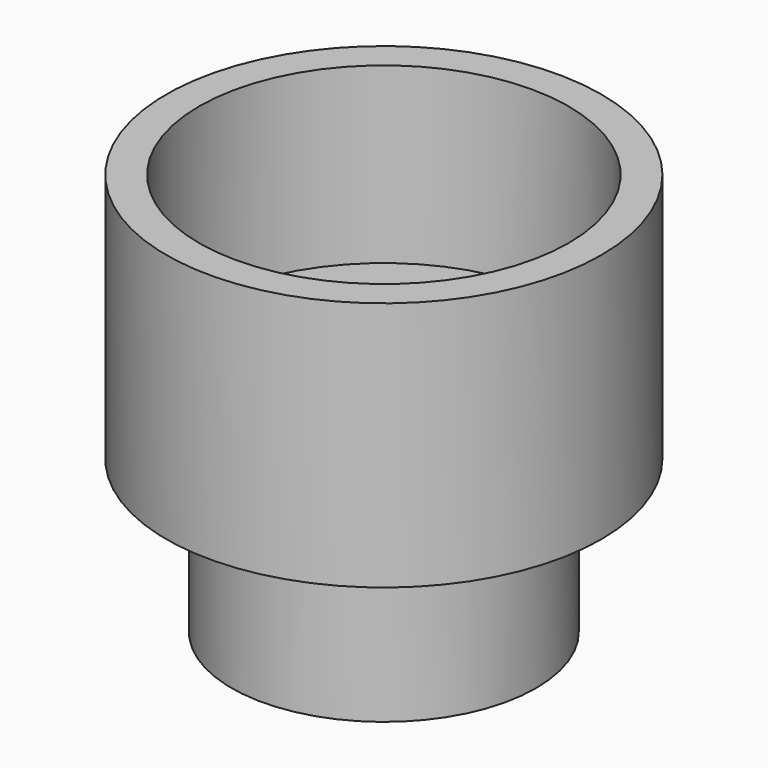
from build123d import *

# Parameters (mm, degrees)
F0_R     = 7
F1_DEPTH = 7
F2_R     = 10
F2_R_2   = 8.5
F2_R_3   = 7
F3_DEPTH = 3.5
F4_R     = 10
F4_R_2   = 8.5
F5_DEPTH = 8


with BuildPart() as f1:
    # F0 (on Top) → F1 (new body)
    with BuildSketch(Plane.XY):
        Circle(F0_R)
        with BuildLine():
            ThreePointArc((-4.2426406871, 1.5), (0, 4.5), (4.2426406871, 1.5))
            Line((4.2426406871, 1.5), (6, 1.5))
            Line((6, 1.5), (6, 0))
            Line((6, 0), (6, -1.5))
            Line((6, -1.5), (4.2426406871, -1.5))
            ThreePointArc((4.2426406871, -1.5), (0, -4.5), (-4.2426406871, -1.5))
            Line((-4.2426406871, -1.5), (-6, -1.5))
            Line((-6, -1.5), (-6, 0))
            Line((-6, 0), (-6, 1.5))
            Line((-6, 1.5), (-4.2426406871, 1.5))
        make_face(mode=Mode.SUBTRACT)
    extrude(amount=F1_DEPTH)

    # F2 (on face) → F3 (join)
    with BuildSketch(Plane.XY.offset(7)):
        Circle(F2_R)
        Circle(F2_R_2, mode=Mode.SUBTRACT)
        Circle(F2_R_2)
        Circle(F2_R_3, mode=Mode.SUBTRACT)
        Circle(F2_R_3)
        with BuildLine():
            Line((-6, 1.5), (-4.2426406871, 1.5))
            ThreePointArc((-4.2426406871, 1.5), (0, 4.5), (4.2426406871, 1.5))
            Line((4.2426406871, 1.5), (6, 1.5))
            Line((6, 1.5), (6, -1.5))
            Line((6, -1.5), (4.2426406871, -1.5))
            ThreePointArc((4.2426406871, -1.5), (0, -4.5), (-4.2426406871, -1.5))
            Line((-4.2426406871, -1.5), (-6, -1.5))
            Line((-6, -1.5), (-6, 1.5))
        make_face(mode=Mode.SUBTRACT)
        with BuildLine():
            ThreePointArc((4.2426406871, 1.5), (0, 4.5), (-4.2426406871, 1.5))
            Line((-4.2426406871, 1.5), (-6, 1.5))
            Line((-6, 1.5), (-6, -1.5))
            Line((-6, -1.5), (-4.2426406871, -1.5))
            ThreePointArc((-4.2426406871, -1.5), (0, -4.5), (4.2426406871, -1.5))
            Line((4.2426406871, -1.5), (6, -1.5))
            Line((6, -1.5), (6, 1.5))
            Line((6, 1.5), (4.2426406871, 1.5))
        make_face()
    extrude(amount=F3_DEPTH)

    # F4 (on face) → F5 (join)
    with BuildSketch(Plane.XY.offset(10.5)):
        Circle(F4_R)
        Circle(F4_R_2, mode=Mode.SUBTRACT)
    extrude(amount=F5_DEPTH)


solid = f1.part
